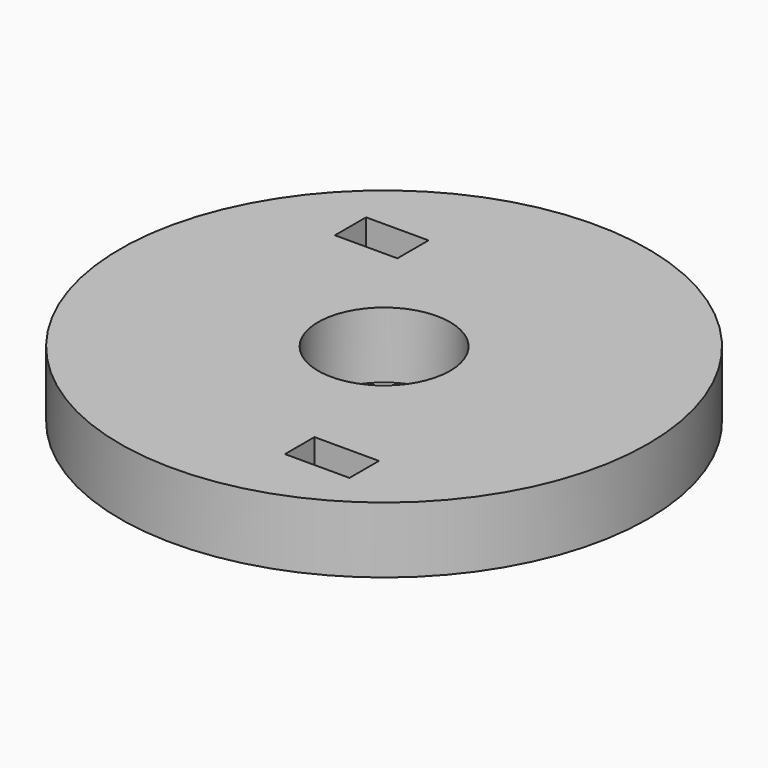
from build123d import *

# Parameters (mm, degrees)
F0_R     = 50.8
F0_R_2   = 12.7
F0_W     = 12.4153457582
F0_H     = 7.0944800973
F0_W_2   = 12.021208182
F0_H_2   = 7.4886232615
F1_DEPTH = 6.35


# Not quite as in the source:
# - a length typed as a fraction of an inch, garbled in the dataset ("3 / 203.2 mm" for 3/8 in), is restored


with BuildPart() as f1:
    # F0 (on Top) → F1 (new body, symmetric)
    with BuildSketch(Plane.XY):
        Circle(F0_R)
        Circle(F0_R_2, mode=Mode.SUBTRACT)
        with Locations((16.4552591741, -33.107586205)):
            Rectangle(F0_W, F0_H, mode=Mode.SUBTRACT)
        with Locations((-22.3673274741, 27.3925866932)):
            Rectangle(F0_W_2, F0_H_2, mode=Mode.SUBTRACT)
    extrude(amount=F1_DEPTH, both=True)


solid = f1.part
